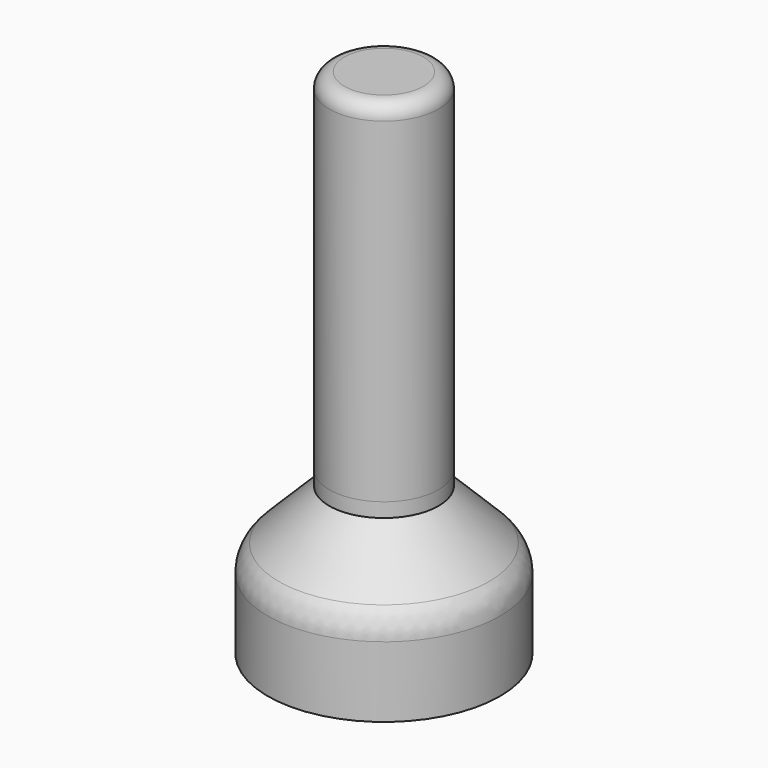
from build123d import *

# Parameters (mm, degrees)
F0_R        = 7.2334484139
F1_DEPTH    = 67.7
F2_R        = 15.3458789883
F3_DEPTH    = 21.4
F4_R        = 2
F5_S5_R     = 7.2334484139
F5_T6_DEPTH = 24
F6_R        = 5


# Not quite as in the source:
# - a fillet or chamfer that OpenCascade refuses, or shapes differently, is made with other operations: its cross-section is extruded or revolved along the edge and cut away or added


with BuildPart() as f1:
    # F0 (on Top) → F1 (new body)
    with BuildSketch(Plane.XY):
        Circle(F0_R)
    extrude(amount=F1_DEPTH)

    # F2 (on Top) → F3 (join)
    with BuildSketch(Plane.XY):
        Circle(F2_R)
    extrude(amount=F3_DEPTH)

    # F4
    f4_edges = [f1.edges().sort_by_distance(p)[0] for p in [
        (-7.233448, 0, 67.7),
    ]]
    fillet(f4_edges, radius=F4_R)

    # F5: chamfer of 10 on 1 edges, made by hand


with BuildPart() as f5_tool2:
    # F5_s3 → F5_t4 (revolve)
    with BuildSketch(Plane.XZ):
        Polygon((5.3458789883, 21.4), (15.3458789883, 11.4), (15.3458789883, 21.4), align=None)
    revolve(axis=Axis((0, 0, 21.4), (0, 0, 1)))

    # F5_s5 → F5_t6 (cut, symmetric)
    with BuildSketch(Plane.XY.offset(16.4)):
        Circle(F5_S5_R)
    extrude(amount=F5_T6_DEPTH, both=True, mode=Mode.SUBTRACT)


with BuildPart() as f1_1:
    add(f1.part)

    # F5_t1: cut F5_tool2
    add(f5_tool2.part, mode=Mode.SUBTRACT)

    # F6
    f6_edges = [f1_1.edges().sort_by_distance(p)[0] for p in [
        (-15.345879, 0, 11.4),
    ]]
    fillet(f6_edges, radius=F6_R)


solid = f1_1.part
